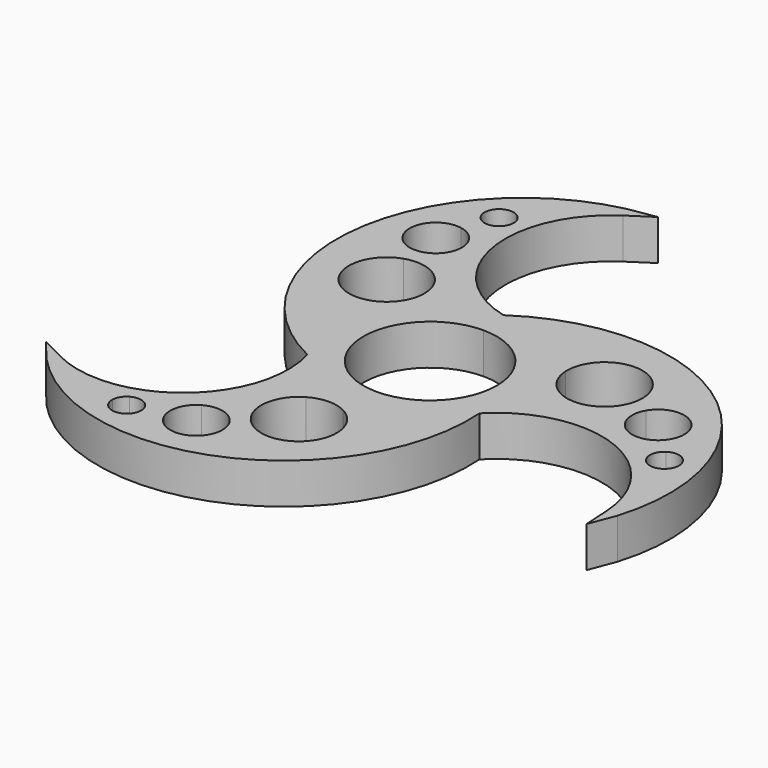
from build123d import *

# Parameters (mm, degrees)
F1_DEPTH = 7
F4_DEPTH = 25
F5_DEPTH = 25
F6_DEPTH = 25
F7_COUNT = 3
F8_DEPTH = 7


# Not quite as in the source:
# - a feature names something its author has since deleted; it is built from what else it names


with BuildPart() as f1:
    # F0 (on Top) → F1 (new body)
    with BuildSketch(Plane.XY):
        with BuildLine():
            ThreePointArc((-13.7992422924, -9.0114684358), (-14.4938657477, 7.8456043045), (0, 16.4810694803))
            ThreePointArc((0, 16.4810694803), (-14.068080809, 30.8723339162), (-6.2153203117, 49.4021353799))
            Line((-6.2153203117, 49.4021353799), (-2.3028528943, 51.9794964298))
            Line((-2.3028528943, 51.9794964298), (-7.0776391154, 51.2091623618))
            ThreePointArc((-7.0776391154, 51.2091623618), (-31.8683563703, 23.4907745685), (-13.7992422924, -9.0114684358))
        make_face()
    extrude(amount=F1_DEPTH)

    # F2 (on Top) → F4 (cut)
    with BuildSketch(Plane.XY):
        with BuildLine():
            ThreePointArc((-19.9399101365, 36.2145881717), (-17.5331910144, 36.3619404524), (-16.370389089, 38.4742617607))
            ThreePointArc((-16.370389089, 38.4742617607), (-16.6966666914, 39.7091427016), (-17.5903338395, 40.6216924484))
            ThreePointArc((-17.5903338395, 40.6216924484), (-18.870389089, 38.4742617607), (-19.9399101365, 36.2145881717))
        make_face()
        with BuildLine():
            ThreePointArc((-12.9184592818, 14.9145969957), (-15.6103285505, 20.1822473574), (-21.4563486152, 21.0868742954))
            ThreePointArc((-21.4563486152, 21.0868742954), (-19.4184592818, 14.9145969957), (-15.9236151324, 9.4340801978))
            ThreePointArc((-15.9236151324, 9.4340801978), (-13.7190519893, 11.7894159586), (-12.9184592818, 14.9145969957))
        make_face()
        with BuildLine():
            ThreePointArc((-15.9236151324, 9.4340801978), (-19.4184592818, 14.9145969957), (-21.4563486152, 21.0868742954))
            ThreePointArc((-21.4563486152, 21.0868742954), (-25.2902206788, 12.1266913129), (-15.9236151324, 9.4340801978))
        make_face()
        with BuildLine():
            ThreePointArc((-17.3422204011, 28.5281271909), (-18.3916105886, 31.4166028999), (-21.0503501441, 32.9579061352))
            ThreePointArc((-21.0503501441, 32.9579061352), (-21.8422204011, 28.5281271909), (-21.8642642373, 24.0281811835))
            ThreePointArc((-21.8642642373, 24.0281811835), (-18.6680431268, 25.3383625238), (-17.3422204011, 28.5281271909))
        make_face()
        with BuildLine():
            ThreePointArc((-21.8642642373, 24.0281811835), (-21.8422204011, 28.5281271909), (-21.0503501441, 32.9579061352))
            ThreePointArc((-21.0503501441, 32.9579061352), (-26.3236437362, 28.9365937035), (-21.8642642373, 24.0281811835))
        make_face()
        with BuildLine():
            ThreePointArc((-19.9399101365, 36.2145881717), (-18.870389089, 38.4742617607), (-17.5903338395, 40.6216924484))
            ThreePointArc((-17.5903338395, 40.6216924484), (-21.0764541807, 39.6503896496), (-19.9399101365, 36.2145881717))
        make_face()
    extrude(amount=-F4_DEPTH, mode=Mode.SUBTRACT)

    # F2 (on Top) → F5 (cut)
    with BuildSketch(Plane.XY):
        with BuildLine():
            ThreePointArc((-19.9399101365, 36.2145881717), (-17.5331910144, 36.3619404524), (-16.370389089, 38.4742617607))
            ThreePointArc((-16.370389089, 38.4742617607), (-16.6966666914, 39.7091427016), (-17.5903338395, 40.6216924484))
            ThreePointArc((-17.5903338395, 40.6216924484), (-18.870389089, 38.4742617607), (-19.9399101365, 36.2145881717))
        make_face()
        with BuildLine():
            ThreePointArc((-12.9184592818, 14.9145969957), (-15.6103285505, 20.1822473574), (-21.4563486152, 21.0868742954))
            ThreePointArc((-21.4563486152, 21.0868742954), (-19.4184592818, 14.9145969957), (-15.9236151324, 9.4340801978))
            ThreePointArc((-15.9236151324, 9.4340801978), (-13.7190519893, 11.7894159586), (-12.9184592818, 14.9145969957))
        make_face()
        with BuildLine():
            ThreePointArc((-15.9236151324, 9.4340801978), (-19.4184592818, 14.9145969957), (-21.4563486152, 21.0868742954))
            ThreePointArc((-21.4563486152, 21.0868742954), (-25.2902206788, 12.1266913129), (-15.9236151324, 9.4340801978))
        make_face()
        with BuildLine():
            ThreePointArc((-17.3422204011, 28.5281271909), (-18.3916105886, 31.4166028999), (-21.0503501441, 32.9579061352))
            ThreePointArc((-21.0503501441, 32.9579061352), (-21.8422204011, 28.5281271909), (-21.8642642373, 24.0281811835))
            ThreePointArc((-21.8642642373, 24.0281811835), (-18.6680431268, 25.3383625238), (-17.3422204011, 28.5281271909))
        make_face()
        with BuildLine():
            ThreePointArc((-21.8642642373, 24.0281811835), (-21.8422204011, 28.5281271909), (-21.0503501441, 32.9579061352))
            ThreePointArc((-21.0503501441, 32.9579061352), (-26.3236437362, 28.9365937035), (-21.8642642373, 24.0281811835))
        make_face()
        with BuildLine():
            ThreePointArc((-19.9399101365, 36.2145881717), (-18.870389089, 38.4742617607), (-17.5903338395, 40.6216924484))
            ThreePointArc((-17.5903338395, 40.6216924484), (-21.0764541807, 39.6503896496), (-19.9399101365, 36.2145881717))
        make_face()
    extrude(amount=-F5_DEPTH, mode=Mode.SUBTRACT)

    # F2 (on Top) → F6 (cut)
    with BuildSketch(Plane.XY):
        with BuildLine():
            ThreePointArc((-19.9399101365, 36.2145881717), (-17.5331910144, 36.3619404524), (-16.370389089, 38.4742617607))
            ThreePointArc((-16.370389089, 38.4742617607), (-16.6966666914, 39.7091427016), (-17.5903338395, 40.6216924484))
            ThreePointArc((-17.5903338395, 40.6216924484), (-18.870389089, 38.4742617607), (-19.9399101365, 36.2145881717))
        make_face()
        with BuildLine():
            ThreePointArc((-12.9184592818, 14.9145969957), (-15.6103285505, 20.1822473574), (-21.4563486152, 21.0868742954))
            ThreePointArc((-21.4563486152, 21.0868742954), (-19.4184592818, 14.9145969957), (-15.9236151324, 9.4340801978))
            ThreePointArc((-15.9236151324, 9.4340801978), (-13.7190519893, 11.7894159586), (-12.9184592818, 14.9145969957))
        make_face()
        with BuildLine():
            ThreePointArc((-15.9236151324, 9.4340801978), (-19.4184592818, 14.9145969957), (-21.4563486152, 21.0868742954))
            ThreePointArc((-21.4563486152, 21.0868742954), (-25.2902206788, 12.1266913129), (-15.9236151324, 9.4340801978))
        make_face()
        with BuildLine():
            ThreePointArc((-17.3422204011, 28.5281271909), (-18.3916105886, 31.4166028999), (-21.0503501441, 32.9579061352))
            ThreePointArc((-21.0503501441, 32.9579061352), (-21.8422204011, 28.5281271909), (-21.8642642373, 24.0281811835))
            ThreePointArc((-21.8642642373, 24.0281811835), (-18.6680431268, 25.3383625238), (-17.3422204011, 28.5281271909))
        make_face()
        with BuildLine():
            ThreePointArc((-21.8642642373, 24.0281811835), (-21.8422204011, 28.5281271909), (-21.0503501441, 32.9579061352))
            ThreePointArc((-21.0503501441, 32.9579061352), (-26.3236437362, 28.9365937035), (-21.8642642373, 24.0281811835))
        make_face()
        with BuildLine():
            ThreePointArc((-19.9399101365, 36.2145881717), (-18.870389089, 38.4742617607), (-17.5903338395, 40.6216924484))
            ThreePointArc((-17.5903338395, 40.6216924484), (-21.0764541807, 39.6503896496), (-19.9399101365, 36.2145881717))
        make_face()
    extrude(amount=F6_DEPTH, mode=Mode.SUBTRACT)


with BuildPart() as f7_1:
    # F7: instance of F1
    add(f1.part.rotate(Axis((0, 0, -1.6987677664), (0, 0, -1)), 1 * 360 / F7_COUNT))


with BuildPart() as f7_2:
    # F7: instance of F1
    add(f1.part.rotate(Axis((0, 0, -1.6987677664), (0, 0, -1)), 2 * 360 / F7_COUNT))


with BuildPart() as f1_1:
    add(f1.part)

    add(f7_1.part)  # F8 merges F7_1

    add(f7_2.part)  # F8 merges F7_2
    # F0 (on Top) → F8 (join)
    with BuildSketch(Plane.XY):
        with BuildLine():
            Line((0, 16.4810694803), (0, 11.5))
            ThreePointArc((0, 11.5), (8.1317279836, 8.1317279836), (11.5, 0))
            ThreePointArc((11.5, 0), (3.2802394095, -11.0222515584), (-9.628700768, -6.2879345989))
            Line((-9.628700768, -6.2879345989), (-13.7992422924, -9.0114684358))
            ThreePointArc((-13.7992422924, -9.0114684358), (4.7010307496, -15.796390762), (16.4810694803, 0))
            ThreePointArc((16.4810694803, 0), (11.6538759907, 11.6538759907), (0, 16.4810694803))
        make_face()
        with BuildLine():
            ThreePointArc((-9.628700768, -6.2879345989), (-10.1133883513, 5.4744292905), (0, 11.5))
            Line((0, 11.5), (0, 16.4810694803))
            ThreePointArc((0, 16.4810694803), (-14.4938657477, 7.8456043045), (-13.7992422924, -9.0114684358))
            Line((-13.7992422924, -9.0114684358), (-9.628700768, -6.2879345989))
        make_face()
    extrude(amount=F8_DEPTH)


solid = f1_1.part
